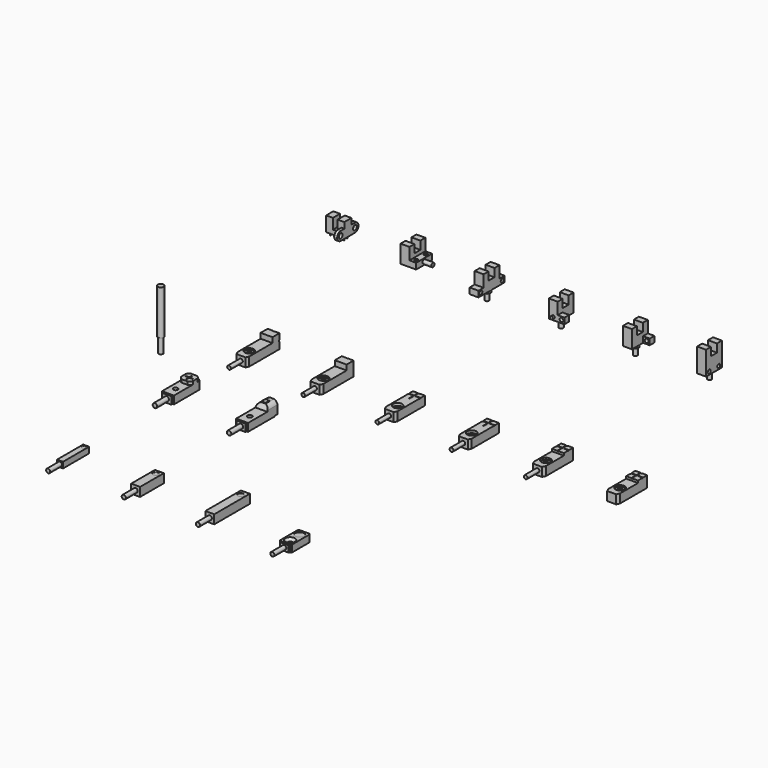
from build123d import *

# Parameters (mm, degrees)
F1_W             = 12.2
F1_H             = 6
F2_DEPTH         = 10
F4_DEPTH         = 2
F5_R             = 1.6
F6_DEPTH         = 2
F7_W             = 3.2
F7_H             = 6
F8_DEPTH         = 7
F9_R             = 0.225
F10_DEPTH        = 2
F11_W            = 6
F11_H            = 13.4
F12_DEPTH        = 12
F13_W            = 6
F13_H            = 5
F14_DEPTH        = 5.5
F15_W            = 13.4
F15_H            = 4
F16_DEPTH        = 4.5
F17_R            = 1.25
F18_DEPTH        = 4
F19_R            = 1.35
F20_DEPTH        = 6
F21_W            = 6
F21_H            = 22
F22_DEPTH        = 4
F23_W            = 6
F23_H            = 13.4
F24_DEPTH        = 8
F25_W            = 6
F25_H            = 5
F26_DEPTH        = 5.5
F27_R            = 1.25
F28_DEPTH        = 6
F29_R            = 2.4
F30_DEPTH        = 2
F31_R            = 1.35
F32_DEPTH        = 5
F33_W            = 6
F33_H            = 13.4
F34_DEPTH        = 12
F35_W            = 6
F35_H            = 5
F36_DEPTH        = 5.5
F37_W            = 4
F37_H            = 4
F38_DEPTH        = 4.5
F39_R            = 1.25
F40_DEPTH        = 4
F41_R            = 1
F42_DEPTH        = 1.5
F43_R            = 2.25
F44_DEPTH        = 2
F45_R            = 1.35
F46_DEPTH        = 5
F47_W            = 6
F47_H            = 13.4
F48_DEPTH        = 12
F49_W            = 4
F49_H            = 4
F50_DEPTH        = 4.5
F51_W            = 6
F51_H            = 5
F52_DEPTH        = 5.5
F53_R            = 1.3452475809
F54_DEPTH        = 4
F55_R            = 1
F56_DEPTH        = 1.5
F57_R            = 2.25
F58_DEPTH        = 2
F59_R            = 1.35
F60_DEPTH        = 5
F61_W            = 6
F61_H            = 13.4
F62_DEPTH        = 16
F63_R            = 1.25
F64_DEPTH        = 6
F65_W            = 6
F65_H            = 5
F66_DEPTH        = 5.5
F67_R            = 1.35
F68_DEPTH        = 5
F69_R            = 2
F70_DEPTH        = 30
F71_R            = 1.5
F72_DEPTH        = 10
F73_W            = 8
F73_H            = 27.5
F74_DEPTH        = 6
F75_W            = 8
F75_H            = 5.9
F76_DEPTH        = 3.5
F78_D            = 2.8
F78_CBORE_D      = 6.2
F78_CBORE_DEPTH  = 1.2
F79_R            = 1.25
F80_DEPTH        = 10
F82_DEPTH        = 0.2
F84_DEPTH        = 6
F85_W            = 8
F85_H            = 27.5
F86_DEPTH        = 6
F87_W            = 8
F87_H            = 5.9
F88_DEPTH        = 3.5
F90_D            = 2.8
F90_CBORE_D      = 6.2
F90_CBORE_DEPTH  = 1.2
F91_R            = 1.25
F92_DEPTH        = 10
F94_DEPTH        = 0.2
F96_DEPTH        = 6
F97_R            = 1
F98_DEPTH        = 1.6
F99_W            = 8
F99_H            = 25
F100_DEPTH       = 6
F102_D           = 2.8
F102_CBORE_D     = 6.2
F102_CBORE_DEPTH = 1.7
F104_DEPTH       = 0.2
F105_R           = 1.25
F106_DEPTH       = 10
F108_DEPTH       = 6
F109_W           = 8
F109_H           = 25
F110_DEPTH       = 6
F112_D           = 2.8
F112_CBORE_D     = 6.2
F112_CBORE_DEPTH = 1.7
F114_DEPTH       = 0.2
F115_R           = 1.25
F116_DEPTH       = 10
F117_R           = 1
F118_DEPTH       = 1.6
F120_DEPTH       = 6
F121_W           = 8
F121_H           = 25
F122_DEPTH       = 6
F124_D           = 2.8
F124_CBORE_D     = 6.2
F124_CBORE_DEPTH = 1.2
F125_W           = 8
F125_H           = 7.8
F126_DEPTH       = 1.5
F128_DEPTH       = 0.2
F129_R           = 1.25
F130_DEPTH       = 10
F131_W           = 8
F131_H           = 25
F132_DEPTH       = 6
F134_D           = 2.8
F134_CBORE_D     = 6.2
F134_CBORE_DEPTH = 1.2
F135_W           = 8
F135_H           = 7.8
F136_DEPTH       = 1.5
F137_W           = 1
F137_H           = 3.4
F137_H_2         = 1
F137_W_2         = 3.5
F138_DEPTH       = 0.2
F140_DEPTH       = 6
F143_R           = 1
F144_DEPTH       = 1.6
F146_DEPTH       = 6
F147_W           = 8
F147_H           = 23
F148_DEPTH       = 5.3
F149_R           = 1.55
F150_DEPTH       = 5.3
F152_DEPTH       = 2.1
F153_W           = 6.3
F153_H           = 5
F154_DEPTH       = 1
F155_R           = 0.5
F156_DEPTH       = 1
F157_SIZE        = 1.5
F158_R           = 1.5
F159_DEPTH       = 10
F160_W           = 2.2871956487
F160_H           = 0.5
F160_W_2         = 0.4256087026
F160_H_2         = 2.25
F161_DEPTH       = 0.5
F162_W           = 8
F162_H           = 25
F163_DEPTH       = 5.3
F164_R           = 1.55
F165_DEPTH       = 5.3
F166_W           = 8
F166_H           = 8.8
F167_DEPTH       = 3.8
F169_DEPTH       = 8
F170_W           = 6.3
F170_H           = 5
F171_DEPTH       = 1
F172_R           = 1.5
F173_DEPTH       = 10
F175_DEPTH       = 8.4135575465
F176_W           = 2.8722813233
F176_H           = 3.2131578947
F177_DEPTH       = 0.5
F178_R           = 1
F179_DEPTH       = 1
F180_W           = 2.75
F180_H           = 0.5
F180_W_2         = 0.5
F180_H_2         = 2.75
F181_DEPTH       = 0.5
F182_W           = 8
F182_H           = 0.4
F183_DEPTH       = 2.5
F184_W           = 4
F184_H           = 22
F185_DEPTH       = 4
F186_R           = 1.4
F187_DEPTH       = 10
F188_R           = 1.5
F189_DEPTH       = 0.2
F190_W           = 6
F190_H           = 20
F191_DEPTH       = 6
F192_R           = 1.4
F193_DEPTH       = 10
F194_R           = 2
F195_DEPTH       = 0.2
F196_W           = 6
F196_H           = 30
F197_DEPTH       = 6
F198_R           = 1.4
F199_DEPTH       = 10
F200_R           = 2
F201_DEPTH       = 0.2
F202_W           = 8
F202_H           = 16
F203_DEPTH       = 4.7
F204_R           = 3
F205_DEPTH       = 0.2
F207_D           = 3.1
F207_CSINK_D     = 6.5
F207_CSINK_ANGLE = 90
F208_W           = 6
F208_H           = 4.3
F209_DEPTH       = 1
F210_R           = 1.4
F211_DEPTH       = 10
F212_SIZE        = 0.5


# Not quite as in the source:
# - the program builds the solid bodies; features that only make, move or delete a surface that nothing else refers to are left out


with BuildPart() as f2:
    # F1 (on Top) → F2 (new body)
    with BuildSketch(Plane.XY):
        Rectangle(F1_W, F1_H)
    extrude(amount=F2_DEPTH)

    # F3 (on face) → F4 (join)
    with BuildSketch(Plane.YZ.offset(6.1)):
        with BuildLine():
            ThreePointArc((6, 0), (9, 3), (6, 6))
            Line((6, 6), (-6, 6))
            ThreePointArc((-6, 6), (-9, 3), (-6, 0))
            Line((-6, 0), (6, 0))
        make_face()
    extrude(amount=-F4_DEPTH)

    # F5 (on face) → F6 (cut, through all)
    with BuildSketch(Plane.YZ.offset(6.1)):
        with Locations((-6, 3)):
            Circle(F5_R)
        with Locations((6, 3)):
            Circle(F5_R)
    extrude(amount=-F6_DEPTH, mode=Mode.SUBTRACT)

    # F7 (on face) → F8 (cut)
    with BuildSketch(Plane.XY.offset(10)):
        Rectangle(F7_W, F7_H)
    extrude(amount=-F8_DEPTH, mode=Mode.SUBTRACT)

    # F9 (on face) → F10 (join)
    with BuildSketch(Plane(origin=(0, 0, 0), x_dir=(1, 0, 0), z_dir=(0, 0, -1))):
        with Locations((-4.6, 1.27)):
            Circle(F9_R)
        with Locations((4.6, 1.27)):
            Circle(F9_R)
        with Locations((4.6, -1.27)):
            Circle(F9_R)
        with Locations((-4.6, -1.27)):
            Circle(F9_R)
    extrude(amount=F10_DEPTH)


with BuildPart() as f12:
    # F11 (on Top) → F12 (new body)
    with BuildSketch(Plane.XY):
        with Locations((50, 0)):
            Rectangle(F11_W, F11_H)
    extrude(amount=F12_DEPTH)

    # F13 (on face) → F14 (cut)
    with BuildSketch(Plane.XY.offset(12)):
        with Locations((50, 0)):
            Rectangle(F13_W, F13_H)
    extrude(amount=-F14_DEPTH, mode=Mode.SUBTRACT)

    # F15 (on face) → F16 (join)
    with BuildSketch(Plane.YZ.offset(53)):
        with Locations((0, 2)):
            Rectangle(F15_W, F15_H)
    extrude(amount=F16_DEPTH)

    # F17 (on face) → F18 (cut, through all)
    with BuildSketch(Plane.XY.offset(4)):
        with Locations((55.5, -4)):
            Circle(F17_R)
        with Locations((55.5, 4)):
            Circle(F17_R)
    extrude(amount=-F18_DEPTH, mode=Mode.SUBTRACT)

    # F19 (on face) → F20 (join)
    with BuildSketch(Plane.YZ.offset(57.5)):
        with Locations((0, 2)):
            Circle(F19_R)
    extrude(amount=F20_DEPTH)


with BuildPart() as f22:
    # F21 (on Top) → F22 (new body)
    with BuildSketch(Plane.XY):
        with Locations((100, 0)):
            Rectangle(F21_W, F21_H)
    extrude(amount=F22_DEPTH)

    # F23 (on face) → F24 (join)
    with BuildSketch(Plane.XY.offset(4)):
        with Locations((100, 0)):
            Rectangle(F23_W, F23_H)
    extrude(amount=F24_DEPTH)

    # F25 (on face) → F26 (cut)
    with BuildSketch(Plane.XY.offset(12)):
        with Locations((100, 0)):
            Rectangle(F25_W, F25_H)
    extrude(amount=-F26_DEPTH, mode=Mode.SUBTRACT)

    # F27 (on face) → F28 (cut, through all)
    with BuildSketch(Plane.YZ.offset(103)):
        with Locations((-9, 2)):
            Circle(F27_R)
        with Locations((9, 2)):
            Circle(F27_R)
    extrude(amount=-F28_DEPTH, mode=Mode.SUBTRACT)

    # F29 (on face) → F30 (join)
    with BuildSketch(Plane(origin=(0, 0, 0), x_dir=(1, 0, 0), z_dir=(0, 0, -1))):
        with Locations((100, 0)):
            Circle(F29_R)
    extrude(amount=F30_DEPTH)

    # F31 (on face) → F32 (join)
    with BuildSketch(Plane(origin=(0, 0, -2), x_dir=(1, 0, 0), z_dir=(0, 0, -1))):
        with Locations((100, 0)):
            Circle(F31_R)
    extrude(amount=F32_DEPTH)


with BuildPart() as f34:
    # F33 (on Top) → F34 (new body)
    with BuildSketch(Plane.XY):
        with Locations((150, 0)):
            Rectangle(F33_W, F33_H)
    extrude(amount=F34_DEPTH)

    # F35 (on face) → F36 (cut)
    with BuildSketch(Plane.XY.offset(12)):
        with Locations((150, 0)):
            Rectangle(F35_W, F35_H)
    extrude(amount=-F36_DEPTH, mode=Mode.SUBTRACT)

    # F37 (on face) → F38 (join)
    with BuildSketch(Plane.YZ.offset(153)):
        with Locations((-4.7, 2)):
            Rectangle(F37_W, F37_H)
    extrude(amount=F38_DEPTH)

    # F39 (on face) → F40 (cut, through all)
    with BuildSketch(Plane.XZ.offset(6.7)):
        with Locations((155.5, 2)):
            Circle(F39_R)
    extrude(amount=-F40_DEPTH, mode=Mode.SUBTRACT)

    # F41 (on face) → F42 (join)
    with BuildSketch(Plane.XZ.offset(6.7)):
        with Locations((150, 2)):
            Circle(F41_R)
    extrude(amount=F42_DEPTH)

    # F43 (on face) → F44 (join)
    with BuildSketch(Plane(origin=(0, 0, 0), x_dir=(1, 0, 0), z_dir=(0, 0, -1))):
        with Locations((150, 0)):
            Circle(F43_R)
    extrude(amount=F44_DEPTH)

    # F45 (on face) → F46 (join)
    with BuildSketch(Plane(origin=(0, 0, -2), x_dir=(1, 0, 0), z_dir=(0, 0, -1))):
        with Locations((150, 0)):
            Circle(F45_R)
    extrude(amount=F46_DEPTH)


with BuildPart() as f48:
    # F47 (on Top) → F48 (new body)
    with BuildSketch(Plane.XY):
        with Locations((200, 0)):
            Rectangle(F47_W, F47_H)
    extrude(amount=F48_DEPTH)

    # F49 (on face) → F50 (join)
    with BuildSketch(Plane.YZ.offset(203)):
        with Locations((4.7, 2)):
            Rectangle(F49_W, F49_H)
    extrude(amount=F50_DEPTH)

    # F51 (on face) → F52 (cut)
    with BuildSketch(Plane.XY.offset(12)):
        with Locations((200, 0)):
            Rectangle(F51_W, F51_H)
    extrude(amount=-F52_DEPTH, mode=Mode.SUBTRACT)

    # F53 (on face) → F54 (cut, through all)
    with BuildSketch(Plane(origin=(0, 6.7, 0), x_dir=(-1, 0, 0), z_dir=(0, 1, 0))):
        with Locations((-205.5, 2)):
            Circle(F53_R)
    extrude(amount=-F54_DEPTH, mode=Mode.SUBTRACT)

    # F55 (on face) → F56 (join)
    with BuildSketch(Plane(origin=(0, 6.7, 0), x_dir=(-1, 0, 0), z_dir=(0, 1, 0))):
        with Locations((-200, 2)):
            Circle(F55_R)
    extrude(amount=F56_DEPTH)

    # F57 (on face) → F58 (join)
    with BuildSketch(Plane(origin=(0, 0, 0), x_dir=(1, 0, 0), z_dir=(0, 0, -1))):
        with Locations((200, 0)):
            Circle(F57_R)
    extrude(amount=F58_DEPTH)

    # F59 (on face) → F60 (join)
    with BuildSketch(Plane(origin=(0, 0, -2), x_dir=(1, 0, 0), z_dir=(0, 0, -1))):
        with Locations((200, 0)):
            Circle(F59_R)
    extrude(amount=F60_DEPTH)


with BuildPart() as f62:
    # F61 (on Top) → F62 (new body)
    with BuildSketch(Plane.XY):
        with Locations((250, 0)):
            Rectangle(F61_W, F61_H)
    extrude(amount=F62_DEPTH)

    # F63 (on face) → F64 (cut, through all)
    with BuildSketch(Plane.YZ.offset(253)):
        with Locations((-4, 2)):
            Circle(F63_R)
        with Locations((4, 2)):
            Circle(F63_R)
    extrude(amount=-F64_DEPTH, mode=Mode.SUBTRACT)

    # F65 (on face) → F66 (cut)
    with BuildSketch(Plane.XY.offset(16)):
        with Locations((250, 0)):
            Rectangle(F65_W, F65_H)
    extrude(amount=-F66_DEPTH, mode=Mode.SUBTRACT)

    # F67 (on face) → F68 (join)
    with BuildSketch(Plane(origin=(0, 0, 0), x_dir=(1, 0, 0), z_dir=(0, 0, -1))):
        with Locations((250, 0)):
            Circle(F67_R)
    extrude(amount=F68_DEPTH)


with BuildPart() as f70:
    # F69 (on Top) → F70 (new body)
    with BuildSketch(Plane.XY):
        with Locations((0, -150)):
            Circle(F69_R)
    extrude(amount=F70_DEPTH)

    # F71 (on face) → F72 (join)
    with BuildSketch(Plane(origin=(0, 0, 0), x_dir=(1, 0, 0), z_dir=(0, 0, -1))):
        with Locations((0, 150)):
            Circle(F71_R)
    extrude(amount=F72_DEPTH)


with BuildPart() as f74:
    # F73 (on Top) → F74 (new body)
    with BuildSketch(Plane.XY):
        with Locations((54, -136.25)):
            Rectangle(F73_W, F73_H)
    extrude(amount=F74_DEPTH)

    # F75 (on face) → F76 (join)
    with BuildSketch(Plane.XY.offset(6)):
        with Locations((54, -125.45)):
            Rectangle(F75_W, F75_H)
    extrude(amount=F76_DEPTH)

    # F78 (through all)
    with Locations(Plane.XY.offset(6)):
        with Locations((54, -142.9)):
            CounterBoreHole(F78_D / 2, F78_CBORE_D / 2, F78_CBORE_DEPTH)

    # F79 (on face) → F80 (join)
    with BuildSketch(Plane.XZ.offset(150)):
        with Locations((54, 3)):
            Circle(F79_R)
    extrude(amount=F80_DEPTH)

    # F81 (on face) → F82 (cut)
    with BuildSketch(Plane(origin=(0, -122.5, 0), x_dir=(-1, 0, 0), z_dir=(0, 1, 0))):
        Polygon((-53.5, 5.4), (-53.5, 9.5), (-54.5, 9.5), (-54.5, 5.4), (-58, 5.4), (-58, 4.4), (-54.5, 4.4), (-54.5, 0), (-53.5, 0), (-53.5, 4.4), (-50, 4.4), (-50, 5.4), align=None)
    extrude(amount=-F82_DEPTH, mode=Mode.SUBTRACT)

    # F83 (on face) → F84 (cut, through all)
    with BuildSketch(Plane.XY.offset(6)):
        Polygon((50, -148), (50, -150), (51, -150), align=None)
        Polygon((58, -150), (58, -148), (57, -150), align=None)
    extrude(amount=-F84_DEPTH, mode=Mode.SUBTRACT)


with BuildPart() as f86:
    # F85 (on Top) → F86 (new body)
    with BuildSketch(Plane.XY):
        with Locations((104, -136.25)):
            Rectangle(F85_W, F85_H)
    extrude(amount=F86_DEPTH)

    # F87 (on face) → F88 (join)
    with BuildSketch(Plane.XY.offset(6)):
        with Locations((104, -125.45)):
            Rectangle(F87_W, F87_H)
    extrude(amount=F88_DEPTH)

    # F90 (through all)
    with Locations(Plane.XY.offset(6)):
        with Locations((104, -142.9)):
            CounterBoreHole(F90_D / 2, F90_CBORE_D / 2, F90_CBORE_DEPTH)

    # F91 (on face) → F92 (join)
    with BuildSketch(Plane.XZ.offset(150)):
        with Locations((104, 3)):
            Circle(F91_R)
    extrude(amount=F92_DEPTH)

    # F93 (on face) → F94 (cut)
    with BuildSketch(Plane(origin=(0, -122.5, 0), x_dir=(-1, 0, 0), z_dir=(0, 1, 0))):
        Polygon((-104.5, 0), (-103.5, 0), (-103.5, 4.4), (-100, 4.4), (-100, 5.4), (-103.5, 5.4), (-103.5, 9.5), (-104.5, 9.5), (-104.5, 5.4), (-108, 5.4), (-108, 4.4), (-104.5, 4.4), align=None)
    extrude(amount=-F94_DEPTH, mode=Mode.SUBTRACT)

    # F95 (on face) → F96 (cut, through all)
    with BuildSketch(Plane.XY.offset(6)):
        Polygon((101, -150), (100, -148), (100, -150), align=None)
        Polygon((108, -150), (108, -148), (107, -150), align=None)
    extrude(amount=-F96_DEPTH, mode=Mode.SUBTRACT)

    # F97 (on face) → F98 (join)
    with BuildSketch(Plane(origin=(0, 0, 0), x_dir=(1, 0, 0), z_dir=(0, 0, -1))):
        with Locations((104, 128.9)):
            Circle(F97_R)
    extrude(amount=F98_DEPTH)


with BuildPart() as f100:
    # F99 (on Top) → F100 (new body)
    with BuildSketch(Plane.XY):
        with Locations((154, -137.5)):
            Rectangle(F99_W, F99_H)
    extrude(amount=F100_DEPTH)

    # F102 (through all)
    with Locations(Plane.XY.offset(6)):
        with Locations((154, -142.9)):
            CounterBoreHole(F102_D / 2, F102_CBORE_D / 2, F102_CBORE_DEPTH)

    # F103 (on face) → F104 (cut)
    with BuildSketch(Plane.XY.offset(6)):
        Polygon((154.5, -125), (153.5, -125), (153.5, -128.4), (150, -128.4), (150, -129.4), (153.5, -129.4), (153.5, -133), (154.5, -133), (154.5, -129.4), (158, -129.4), (158, -128.4), (154.5, -128.4), align=None)
    extrude(amount=-F104_DEPTH, mode=Mode.SUBTRACT)

    # F105 (on face) → F106 (join)
    with BuildSketch(Plane.XZ.offset(150)):
        with Locations((154, 3)):
            Circle(F105_R)
    extrude(amount=F106_DEPTH)

    # F107 (on face) → F108 (cut, through all)
    with BuildSketch(Plane.XY.offset(6)):
        Polygon((151, -150), (150, -148), (150, -150), align=None)
        Polygon((158, -150), (158, -148), (157, -150), align=None)
    extrude(amount=-F108_DEPTH, mode=Mode.SUBTRACT)


with BuildPart() as f110:
    # F109 (on Top) → F110 (new body)
    with BuildSketch(Plane.XY):
        with Locations((204, -137.5)):
            Rectangle(F109_W, F109_H)
    extrude(amount=F110_DEPTH)

    # F112 (through all)
    with Locations(Plane.XY.offset(6)):
        with Locations((204, -142.9)):
            CounterBoreHole(F112_D / 2, F112_CBORE_D / 2, F112_CBORE_DEPTH)

    # F113 (on face) → F114 (cut)
    with BuildSketch(Plane.XY.offset(6)):
        Polygon((204.5, -125), (203.5, -125), (203.5, -128.4), (200, -128.4), (200, -129.4), (203.5, -129.4), (203.5, -133), (204.5, -133), (204.5, -129.4), (208, -129.4), (208, -128.4), (204.5, -128.4), align=None)
    extrude(amount=-F114_DEPTH, mode=Mode.SUBTRACT)

    # F115 (on face) → F116 (join)
    with BuildSketch(Plane.XZ.offset(150)):
        with Locations((204, 3)):
            Circle(F115_R)
    extrude(amount=F116_DEPTH)

    # F117 (on face) → F118 (join)
    with BuildSketch(Plane(origin=(0, 0, 0), x_dir=(1, 0, 0), z_dir=(0, 0, -1))):
        with Locations((204, 128.9)):
            Circle(F117_R)
    extrude(amount=F118_DEPTH)

    # F119 (on face) → F120 (cut, through all)
    with BuildSketch(Plane.XY.offset(6)):
        Polygon((201, -150), (200, -148), (200, -150), align=None)
        Polygon((208, -150), (208, -148), (207, -150), align=None)
    extrude(amount=-F120_DEPTH, mode=Mode.SUBTRACT)


with BuildPart() as f122:
    # F121 (on Top) → F122 (new body)
    with BuildSketch(Plane.XY):
        with Locations((254, -137.5)):
            Rectangle(F121_W, F121_H)
    extrude(amount=F122_DEPTH)

    # F124 (through all)
    with Locations(Plane.XY.offset(6)):
        with Locations((254, -142.9)):
            CounterBoreHole(F124_D / 2, F124_CBORE_D / 2, F124_CBORE_DEPTH)

    # F125 (on face) → F126 (join)
    with BuildSketch(Plane.XY.offset(6)):
        with Locations((254, -128.9)):
            Rectangle(F125_W, F125_H)
    extrude(amount=F126_DEPTH)

    # F127 (on face) → F128 (cut)
    with BuildSketch(Plane.XY.offset(7.5)):
        Polygon((254.5, -125), (253.5, -125), (253.5, -128.4), (250, -128.4), (250, -129.4), (253.5, -129.4), (253.5, -132.8), (254.5, -132.8), (254.5, -129.4), (258, -129.4), (258, -128.4), (254.5, -128.4), align=None)
    extrude(amount=-F128_DEPTH, mode=Mode.SUBTRACT)

    # F129 (on face) → F130 (join)
    with BuildSketch(Plane.XZ.offset(150)):
        with Locations((254, 3)):
            Circle(F129_R)
    extrude(amount=F130_DEPTH)

    # F139 (on face) → F140 (cut, through all)
    with BuildSketch(Plane.XY.offset(6)):
        Polygon((251, -150), (250, -148), (250, -150), align=None)
        Polygon((258, -150), (258, -148), (257, -150), align=None)
    extrude(amount=-F140_DEPTH, mode=Mode.SUBTRACT)


with BuildPart() as f132:
    # F131 (on Top) → F132 (new body)
    with BuildSketch(Plane.XY):
        with Locations((304, -137.5)):
            Rectangle(F131_W, F131_H)
    extrude(amount=F132_DEPTH)

    # F134 (through all)
    with Locations(Plane.XY.offset(6)):
        with Locations((304, -142.9)):
            CounterBoreHole(F134_D / 2, F134_CBORE_D / 2, F134_CBORE_DEPTH)

    # F135 (on face) → F136 (join)
    with BuildSketch(Plane.XY.offset(6)):
        with Locations((304, -128.9)):
            Rectangle(F135_W, F135_H)
    extrude(amount=F136_DEPTH)

    # F137 (on face) → F138 (cut)
    with BuildSketch(Plane.XY.offset(7.5)):
        with Locations((304, -126.7)):
            Rectangle(F137_W, F137_H)
        with Locations((304, -128.9)):
            Rectangle(F137_W, F137_H_2)
        with Locations((301.75, -128.9)):
            Rectangle(F137_W_2, F137_H_2)
        with Locations((306.25, -128.9)):
            Rectangle(F137_W_2, F137_H_2)
        with Locations((304, -131.1)):
            Rectangle(F137_W, F137_H)
    extrude(amount=-F138_DEPTH, mode=Mode.SUBTRACT)

    # F143 (on face) → F144 (join)
    with BuildSketch(Plane(origin=(0, 0, 0), x_dir=(1, 0, 0), z_dir=(0, 0, -1))):
        with Locations((304, 128.9)):
            Circle(F143_R)
    extrude(amount=F144_DEPTH)

    # F145 (on face) → F146 (cut, through all)
    with BuildSketch(Plane.XY.offset(6)):
        Polygon((301, -150), (300, -148), (300, -150), align=None)
        Polygon((308, -150), (308, -148), (307, -150), align=None)
    extrude(amount=-F146_DEPTH, mode=Mode.SUBTRACT)


with BuildPart() as f148:
    # F147 (on Top) → F148 (new body)
    with BuildSketch(Plane.XY):
        with Locations((50, -195)):
            Rectangle(F147_W, F147_H)
    extrude(amount=F148_DEPTH)

    # F149 (on face) → F150 (cut, through all)
    with BuildSketch(Plane.XY.offset(5.3)):
        with Locations((50, -200)):
            Circle(F149_R)
    extrude(amount=-F150_DEPTH, mode=Mode.SUBTRACT)

    # F151 (on face) → F152 (join)
    with BuildSketch(Plane.XY.offset(5.3)):
        with BuildLine():
            Line((52.0615528128, -184.5), (47.9384471872, -184.5))
            ThreePointArc((47.9384471872, -184.5), (46.8180194847, -185.3180194847), (46, -186.4384471872))
            Line((46, -186.4384471872), (46, -190.5615528128))
            ThreePointArc((46, -190.5615528128), (46.8180194847, -191.6819805153), (47.9384471872, -192.5))
            Line((47.9384471872, -192.5), (52.0615528128, -192.5))
            ThreePointArc((52.0615528128, -192.5), (53.1819805153, -191.6819805153), (54, -190.5615528128))
            Line((54, -190.5615528128), (54, -186.4384471872))
            ThreePointArc((54, -186.4384471872), (53.1819805153, -185.3180194847), (52.0615528128, -184.5))
        make_face()
    extrude(amount=F152_DEPTH)

    # F153 (on face) → F154 (join)
    with BuildSketch(Plane.XZ.offset(206.5)):
        with Locations((50, 2.5)):
            Rectangle(F153_W, F153_H)
    extrude(amount=F154_DEPTH)

    # F155 (on face) → F156 (cut)
    with BuildSketch(Plane.XY.offset(7.4)):
        with Locations((50, -188.5)):
            Circle(F155_R)
    extrude(amount=-F156_DEPTH, mode=Mode.SUBTRACT)

    # F157
    f157_edges = [f148.edges().sort_by_distance(p)[0] for p in [
        (54, -183.5, 2.65),
        (46, -183.5, 2.65),
    ]]
    chamfer(f157_edges, length=F157_SIZE)

    # F158 (on face) → F159 (join)
    with BuildSketch(Plane.XZ.offset(207.5)):
        with Locations((50, 2.5)):
            Circle(F158_R)
    extrude(amount=F159_DEPTH)

    # F160 (on face) → F161 (cut)
    with BuildSketch(Plane.XY.offset(7.4)):
        with Locations((51.3564021757, -188.5)):
            Rectangle(F160_W, F160_H)
        with Locations((50, -188.5)):
            Rectangle(F160_W_2, F160_H)
        with Locations((50, -187.125)):
            Rectangle(F160_W_2, F160_H_2)
        with Locations((48.6435978243, -188.5)):
            Rectangle(F160_W, F160_H)
        with Locations((50, -189.875)):
            Rectangle(F160_W_2, F160_H_2)
    extrude(amount=-F161_DEPTH, mode=Mode.SUBTRACT)


with BuildPart() as f163:
    # F162 (on Top) → F163 (new body)
    with BuildSketch(Plane.XY):
        with Locations((100, -194)):
            Rectangle(F162_W, F162_H)
    extrude(amount=F163_DEPTH)

    # F164 (on face) → F165 (cut, through all)
    with BuildSketch(Plane.XY.offset(5.3)):
        with Locations((100, -200)):
            Circle(F164_R)
    extrude(amount=-F165_DEPTH, mode=Mode.SUBTRACT)

    # F166 (on face) → F167 (join)
    with BuildSketch(Plane.XY.offset(5.3)):
        with Locations((100, -185.9)):
            Rectangle(F166_W, F166_H)
    extrude(amount=F167_DEPTH)

    # F168 (on face) → F169 (cut, through all)
    with BuildSketch(Plane(origin=(96, 0, 0), x_dir=(0, -1, 0), z_dir=(-1, 0, 0))):
        Polygon((188.3, 9.1), (190.3, 5.3), (190.3, 9.1), align=None)
    extrude(amount=-F169_DEPTH, mode=Mode.SUBTRACT)

    # F170 (on face) → F171 (join)
    with BuildSketch(Plane.XZ.offset(206.5)):
        with Locations((100, 2.5)):
            Rectangle(F170_W, F170_H)
    extrude(amount=F171_DEPTH)

    # F172 (on face) → F173 (join)
    with BuildSketch(Plane.XZ.offset(207.5)):
        with Locations((100, 2.5)):
            Circle(F172_R)
    extrude(amount=F173_DEPTH)

    # F174 (on face) → F175 (cut, through all)
    with BuildSketch(Plane(origin=(0, -181.5, 0), x_dir=(-1, 0, 0), z_dir=(0, 1, 0))):
        with BuildLine():
            ThreePointArc((-98.5638593384, 8.6), (-96.99479618, 7.60520382), (-96, 6.0361406616))
            Line((-96, 6.0361406616), (-96, 9.1))
            Line((-96, 9.1), (-104, 9.1))
            Line((-104, 9.1), (-104, 6.0361406616))
            ThreePointArc((-104, 6.0361406616), (-103.00520382, 7.60520382), (-101.4361406616, 8.6))
            Line((-101.4361406616, 8.6), (-98.5638593384, 8.6))
        make_face()
    extrude(amount=-F175_DEPTH, mode=Mode.SUBTRACT)

    # F176 (on face) → F177 (join)
    with BuildSketch(Plane.XY.offset(8.6)):
        with Locations((100, -186.9565789474)):
            Rectangle(F176_W, F176_H)
    extrude(amount=F177_DEPTH)

    # F178 (on face) → F179 (cut)
    with BuildSketch(Plane(origin=(0, -181.5, 0), x_dir=(-1, 0, 0), z_dir=(0, 1, 0))):
        with Locations((-100, 4.6)):
            Circle(F178_R)
    extrude(amount=-F179_DEPTH, mode=Mode.SUBTRACT)

    # F180 (on face) → F181 (cut)
    with BuildSketch(Plane(origin=(0, -181.5, 0), x_dir=(-1, 0, 0), z_dir=(0, 1, 0))):
        with Locations((-98.375, 4.6)):
            Rectangle(F180_W, F180_H)
        with Locations((-100, 4.6)):
            Rectangle(F180_W_2, F180_H)
        with Locations((-100, 6.225)):
            Rectangle(F180_W_2, F180_H_2)
        with Locations((-101.625, 4.6)):
            Rectangle(F180_W, F180_H)
        with Locations((-100, 2.975)):
            Rectangle(F180_W_2, F180_H_2)
    extrude(amount=-F181_DEPTH, mode=Mode.SUBTRACT)

    # F182 (on face) → F183 (cut)
    with BuildSketch(Plane(origin=(0, -181.5, 0), x_dir=(-1, 0, 0), z_dir=(0, 1, 0))):
        with Locations((-100, 0.2)):
            Rectangle(F182_W, F182_H)
    extrude(amount=-F183_DEPTH, mode=Mode.SUBTRACT)


with BuildPart() as f185:
    # F184 (on Top) → F185 (new body)
    with BuildSketch(Plane.XY):
        with Locations((52, -289)):
            Rectangle(F184_W, F184_H)
    extrude(amount=F185_DEPTH)

    # F186 (on face) → F187 (join)
    with BuildSketch(Plane.XZ.offset(300)):
        with Locations((52, 2)):
            Circle(F186_R)
    extrude(amount=F187_DEPTH)

    # F188 (on face) → F189 (cut)
    with BuildSketch(Plane.XY.offset(4)):
        with Locations((52, -280)):
            Circle(F188_R)
    extrude(amount=-F189_DEPTH, mode=Mode.SUBTRACT)


with BuildPart() as f191:
    # F190 (on Top) → F191 (new body)
    with BuildSketch(Plane.XY):
        with Locations((103, -290)):
            Rectangle(F190_W, F190_H)
    extrude(amount=F191_DEPTH)

    # F192 (on face) → F193 (join)
    with BuildSketch(Plane.XZ.offset(300)):
        with Locations((103, 3)):
            Circle(F192_R)
    extrude(amount=F193_DEPTH)

    # F194 (on face) → F195 (cut)
    with BuildSketch(Plane.XY.offset(6)):
        with Locations((103, -283)):
            Circle(F194_R)
    extrude(amount=-F195_DEPTH, mode=Mode.SUBTRACT)


with BuildPart() as f197:
    # F196 (on Top) → F197 (new body)
    with BuildSketch(Plane.XY):
        with Locations((153, -285)):
            Rectangle(F196_W, F196_H)
    extrude(amount=F197_DEPTH)

    # F198 (on face) → F199 (join)
    with BuildSketch(Plane.XZ.offset(300)):
        with Locations((153, 3)):
            Circle(F198_R)
    extrude(amount=F199_DEPTH)

    # F200 (on face) → F201 (cut)
    with BuildSketch(Plane.XY.offset(6)):
        with Locations((153, -274)):
            Circle(F200_R)
    extrude(amount=-F201_DEPTH, mode=Mode.SUBTRACT)


with BuildPart() as f203:
    # F202 (on Top) → F203 (new body)
    with BuildSketch(Plane.XY):
        with Locations((204, -292)):
            Rectangle(F202_W, F202_H)
    extrude(amount=F203_DEPTH)

    # F204 (on face) → F205 (cut)
    with BuildSketch(Plane.XY.offset(4.7)):
        with Locations((204, -288)):
            Circle(F204_R)
    extrude(amount=-F205_DEPTH, mode=Mode.SUBTRACT)

    # F207 (through all)
    with Locations(Plane.XY.offset(4.7)):
        with Locations((204, -296)):
            CounterSinkHole(F207_D / 2, F207_CSINK_D / 2, counter_sink_angle=F207_CSINK_ANGLE)

    # F208 (on face) → F209 (join)
    with BuildSketch(Plane.XZ.offset(300)):
        with Locations((204, 2.35)):
            Rectangle(F208_W, F208_H)
    extrude(amount=F209_DEPTH)

    # F210 (on face) → F211 (join)
    with BuildSketch(Plane.XZ.offset(301)):
        with Locations((204, 2.35)):
            Circle(F210_R)
    extrude(amount=F211_DEPTH)

    # F212
    f212_edges = [f203.edges().sort_by_distance(p)[0] for p in [
        (208, -284, 2.35),
        (208, -300, 2.35),
        (200, -300, 2.35),
        (200, -284, 2.35),
    ]]
    chamfer(f212_edges, length=F212_SIZE)


solid = Compound([f2.part, f12.part, f22.part, f34.part, f48.part, f62.part, f70.part, f74.part, f86.part, f100.part, f110.part, f122.part, f132.part, f148.part, f163.part, f185.part, f191.part, f197.part, f203.part])
